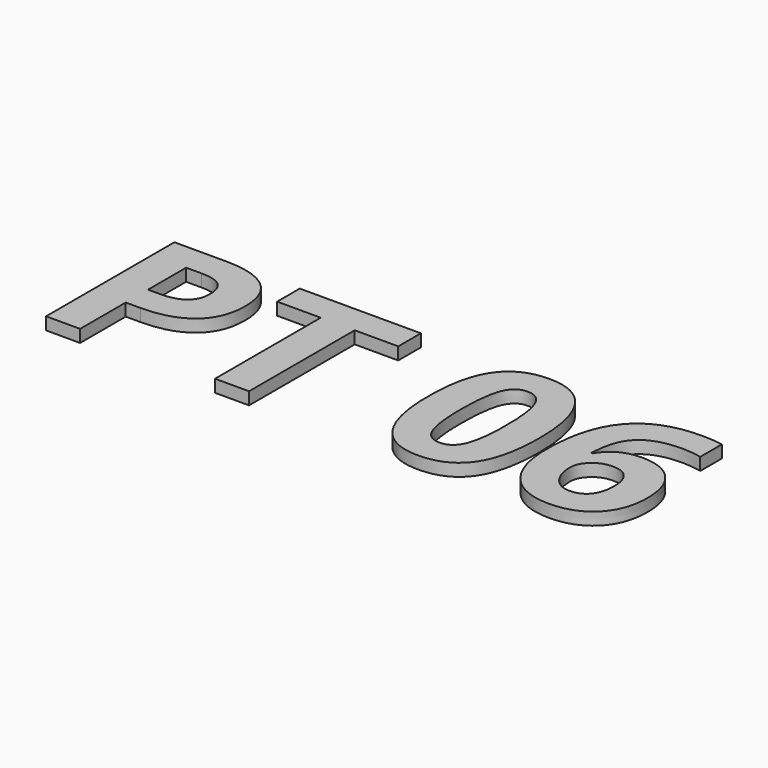
from build123d import *

# Parameters (mm, degrees)
F0_TEXT_SIZE = 18.0555555556
F1_DEPTH     = 1


# Not quite as in the source:
# - Text() gives the source's letters only with a copy of the font that has no kerning and outlines rounded to 1/6400 em; it was checked with that copy


with BuildPart() as f1:
    # F0 (on Top) → F1 (new body)
    with BuildSketch(Plane.XY):
        with Locations((-23.8474392361, -6.5)):
            Text('PT 06', F0_TEXT_SIZE, font='Open Sans', font_style=FontStyle.BOLD, text_align=(TextAlign.LEFT, TextAlign.BOTTOM))
    extrude(amount=F1_DEPTH)


solid = f1.part
